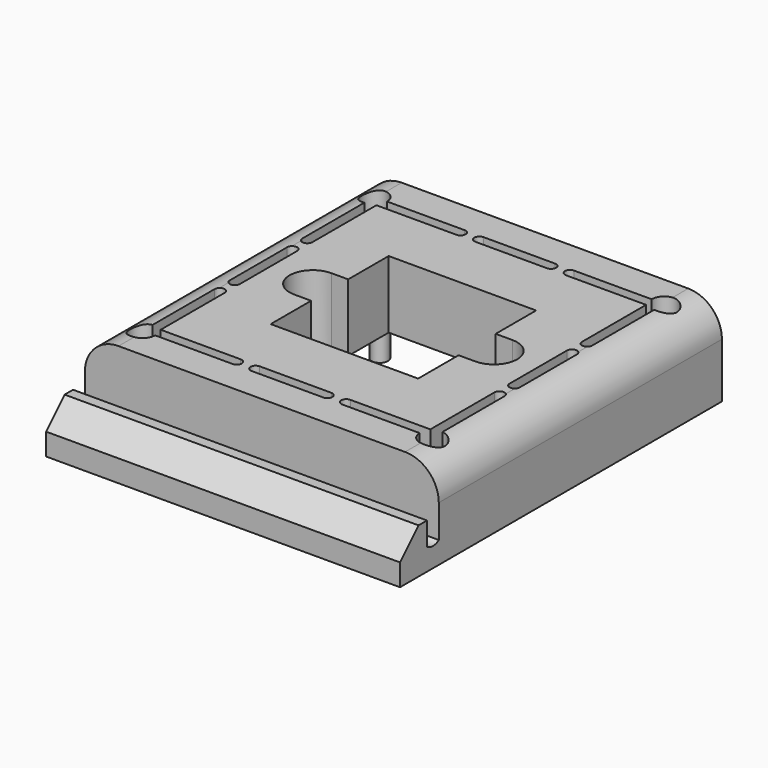
from build123d import *

# Parameters (mm, degrees)
F0_W        = 39
F0_H        = 39
F0_R        = 0.975
F1_DEPTH    = 9
F2_T1_DEPTH = 62
F4_DEPTH    = 21
F5_DEPTH    = 21
F6_DEPTH    = 5.5
F7_DEPTH    = 1.5
F8_DEPTH    = 2.5
F9_DEPTH    = 1.5
F10_R       = 1.25
F11_DEPTH   = 2.5
F12_DEPTH   = 5
F13_DEPTH   = 1


# Not quite as in the source:
# - a fillet or chamfer that OpenCascade refuses, or shapes differently, is made with other operations: its cross-section is extruded or revolved along the edge and cut away or added


with BuildPart() as f1:
    # F0 (on Top) → F1 (new body)
    with BuildSketch(Plane.XY):
        Polygon((-2.625, 21), (-21, 21), (-21, -21), (-2.625, -21), (2.625, -21), (21, -21), (21, 21), (2.625, 21), align=None)
        Rectangle(F0_W, F0_H, mode=Mode.SUBTRACT)
        Rectangle(F0_W, F0_H)
        with BuildLine():
            ThreePointArc((16, 4.25), (16.6, 4.85), (17.2, 4.25))
            Line((17.2, 4.25), (17.2, -4.25))
            ThreePointArc((17.2, -4.25), (16.6, -4.85), (16, -4.25))
            Line((16, -4.25), (16, -6.5))
            ThreePointArc((16, -6.5), (16.6, -5.9), (17.2, -6.5))
            Line((17.2, -6.5), (17.2, -15.7))
            ThreePointArc((17.2, -15.7), (18.2606601718, -18.2606601718), (15.7, -17.2))
            Line((15.7, -17.2), (6.5, -17.2))
            ThreePointArc((6.5, -17.2), (5.9, -16.6), (6.5, -16))
            Line((6.5, -16), (4.25, -16))
            ThreePointArc((4.25, -16), (4.85, -16.6), (4.25, -17.2))
            Line((4.25, -17.2), (-4.25, -17.2))
            ThreePointArc((-4.25, -17.2), (-4.85, -16.6), (-4.25, -16))
            Line((-4.25, -16), (-6.5, -16))
            ThreePointArc((-6.5, -16), (-5.9, -16.6), (-6.5, -17.2))
            Line((-6.5, -17.2), (-15.7, -17.2))
            ThreePointArc((-15.7, -17.2), (-18.2606601718, -18.2606601718), (-17.2, -15.7))
            Line((-17.2, -15.7), (-17.2, -6.5))
            ThreePointArc((-17.2, -6.5), (-16.6, -5.9), (-16, -6.5))
            Line((-16, -6.5), (-16, -4.25))
            ThreePointArc((-16, -4.25), (-16.6, -4.85), (-17.2, -4.25))
            Line((-17.2, -4.25), (-17.2, 4.25))
            ThreePointArc((-17.2, 4.25), (-16.6, 4.85), (-16, 4.25))
            Line((-16, 4.25), (-16, 6.5))
            ThreePointArc((-16, 6.5), (-16.6, 5.9), (-17.2, 6.5))
            Line((-17.2, 6.5), (-17.2, 15.7))
            ThreePointArc((-17.2, 15.7), (-18.2606601718, 18.2606601718), (-15.7, 17.2))
            Line((-15.7, 17.2), (-6.5, 17.2))
            ThreePointArc((-6.5, 17.2), (-5.9, 16.6), (-6.5, 16))
            Line((-6.5, 16), (-4.25, 16))
            ThreePointArc((-4.25, 16), (-4.85, 16.6), (-4.25, 17.2))
            Line((-4.25, 17.2), (4.25, 17.2))
            ThreePointArc((4.25, 17.2), (4.85, 16.6), (4.25, 16))
            Line((4.25, 16), (6.5, 16))
            ThreePointArc((6.5, 16), (5.9, 16.6), (6.5, 17.2))
            Line((6.5, 17.2), (15.7, 17.2))
            ThreePointArc((15.7, 17.2), (18.2606601718, 18.2606601718), (17.2, 15.7))
            Line((17.2, 15.7), (17.2, 6.5))
            ThreePointArc((17.2, 6.5), (16.6, 5.9), (16, 6.5))
            Line((16, 6.5), (16, 4.25))
        make_face(mode=Mode.SUBTRACT)
        Polygon((16, -4.25), (16, 4.25), (16, 6.5), (16, 16), (6.5, 16), (4.25, 16), (-4.25, 16), (-6.5, 16), (-16, 16), (-16, 6.5), (-16, 4.25), (-16, -4.25), (-16, -6.5), (-16, -16), (-6.5, -16), (-4.25, -16), (4.25, -16), (6.5, -16), (16, -16), (16, -6.5), align=None)
        with Locations((-14, -14)):
            Circle(F0_R, mode=Mode.SUBTRACT)
        with Locations((14, -14)):
            Circle(F0_R, mode=Mode.SUBTRACT)
        with Locations((-14, 14)):
            Circle(F0_R, mode=Mode.SUBTRACT)
        Polygon((-8.75, 14), (0, 14), (0, 10.75), (-8.75, 10.75), (-9.75, 10.75), (-9.75, 14), align=None, mode=Mode.SUBTRACT)
        with BuildLine():
            Line((-8.75, 8.75), (8.75, 8.75))
            Line((8.75, 8.75), (8.75, 2.75))
            Line((8.75, 2.75), (10.75, 2.75))
            ThreePointArc((10.75, 2.75), (13.5, 0), (10.75, -2.75))
            Line((10.75, -2.75), (8.75, -2.75))
            Line((8.75, -2.75), (8.75, -8.75))
            Line((8.75, -8.75), (-8.75, -8.75))
            Line((-8.75, -8.75), (-8.75, -2.75))
            Line((-8.75, -2.75), (-10.75, -2.75))
            ThreePointArc((-10.75, -2.75), (-13.5, 0), (-10.75, 2.75))
            Line((-10.75, 2.75), (-8.75, 2.75))
            Line((-8.75, 2.75), (-8.75, 8.75))
        make_face(mode=Mode.SUBTRACT)
        Polygon((10.75, 3.8126846775), (10.75, 8.75), (10.75, 9.75), (14, 9.75), (14, 8.75), (14, 3.8126846775), align=None, mode=Mode.SUBTRACT)
        with Locations((14, 14)):
            Circle(F0_R, mode=Mode.SUBTRACT)
        Polygon((0, 10.75), (0, 14), (-8.75, 14), (-9.75, 14), (-9.75, 10.75), (-8.75, 10.75), align=None)
        Polygon((10.75, 9.75), (10.75, 8.75), (10.75, 3.8126846775), (14, 3.8126846775), (14, 8.75), (14, 9.75), align=None)
        with Locations((14, -14)):
            Circle(F0_R)
        with Locations((-14, -14)):
            Circle(F0_R)
        with Locations((-14, 14)):
            Circle(F0_R)
        with Locations((14, 14)):
            Circle(F0_R)
    extrude(amount=F1_DEPTH)

    # F2: fillet of radius 4 on 2 edges, made by hand

    # F2_s2 → F2_t1 (cut)
    with BuildSketch(Plane.XZ.offset(-31)):
        with BuildLine():
            ThreePointArc((-21, 5), (-19.8284271247, 7.8284271247), (-17, 9))
            Line((-17, 9), (-21, 9))
            Line((-21, 9), (-21, 5))
        make_face()
        with BuildLine():
            ThreePointArc((21, 5), (19.8284271247, 7.8284271247), (17, 9))
            Line((17, 9), (21, 9))
            Line((21, 9), (21, 5))
        make_face()
    extrude(amount=F2_T1_DEPTH, mode=Mode.SUBTRACT)

    # F3 (on Right) → F4 (join)
    with BuildSketch(Plane.YZ):
        with BuildLine():
            Line((-21, 0), (-21, 1.1))
            ThreePointArc((-21, 1.1), (-21.875, 0.8183492931), (-22.75, 1.1))
            Line((-22.75, 1.1), (-22.75, 3.85))
            Line((-22.75, 3.85), (-24, 3.85))
            Line((-24, 3.85), (-26.75, 1.1))
            Line((-26.75, 1.1), (-26.75, -1.5))
            Line((-26.75, -1.5), (-22.75, -1.5))
            Line((-22.75, -1.5), (-21, -1.5))
            Line((-21, -1.5), (-21, 0))
        make_face()
    extrude(amount=F4_DEPTH)

    # F5 (add): a face of the model
    f5_faces = [f1.faces().sort_by_distance(p)[0] for p in [
        (0, -24.00739598, 0.5868334208),
    ]]
    extrude(f5_faces, amount=F5_DEPTH)

    # F0 (on Top) → F6 (join)
    with BuildSketch(Plane.XY):
        with Locations((-14, -14)):
            Circle(F0_R)
        with Locations((14, -14)):
            Circle(F0_R)
        with Locations((-14, 14)):
            Circle(F0_R)
        with Locations((14, 14)):
            Circle(F0_R)
    extrude(amount=-F6_DEPTH)

    # F0 (on Top) → F7 (join)
    with BuildSketch(Plane.XY):
        Rectangle(F0_W, F0_H)
        with BuildLine():
            ThreePointArc((16, 4.25), (16.6, 4.85), (17.2, 4.25))
            Line((17.2, 4.25), (17.2, -4.25))
            ThreePointArc((17.2, -4.25), (16.6, -4.85), (16, -4.25))
            Line((16, -4.25), (16, -6.5))
            ThreePointArc((16, -6.5), (16.6, -5.9), (17.2, -6.5))
            Line((17.2, -6.5), (17.2, -15.7))
            ThreePointArc((17.2, -15.7), (18.2606601718, -18.2606601718), (15.7, -17.2))
            Line((15.7, -17.2), (6.5, -17.2))
            ThreePointArc((6.5, -17.2), (5.9, -16.6), (6.5, -16))
            Line((6.5, -16), (4.25, -16))
            ThreePointArc((4.25, -16), (4.85, -16.6), (4.25, -17.2))
            Line((4.25, -17.2), (-4.25, -17.2))
            ThreePointArc((-4.25, -17.2), (-4.85, -16.6), (-4.25, -16))
            Line((-4.25, -16), (-6.5, -16))
            ThreePointArc((-6.5, -16), (-5.9, -16.6), (-6.5, -17.2))
            Line((-6.5, -17.2), (-15.7, -17.2))
            ThreePointArc((-15.7, -17.2), (-18.2606601718, -18.2606601718), (-17.2, -15.7))
            Line((-17.2, -15.7), (-17.2, -6.5))
            ThreePointArc((-17.2, -6.5), (-16.6, -5.9), (-16, -6.5))
            Line((-16, -6.5), (-16, -4.25))
            ThreePointArc((-16, -4.25), (-16.6, -4.85), (-17.2, -4.25))
            Line((-17.2, -4.25), (-17.2, 4.25))
            ThreePointArc((-17.2, 4.25), (-16.6, 4.85), (-16, 4.25))
            Line((-16, 4.25), (-16, 6.5))
            ThreePointArc((-16, 6.5), (-16.6, 5.9), (-17.2, 6.5))
            Line((-17.2, 6.5), (-17.2, 15.7))
            ThreePointArc((-17.2, 15.7), (-18.2606601718, 18.2606601718), (-15.7, 17.2))
            Line((-15.7, 17.2), (-6.5, 17.2))
            ThreePointArc((-6.5, 17.2), (-5.9, 16.6), (-6.5, 16))
            Line((-6.5, 16), (-4.25, 16))
            ThreePointArc((-4.25, 16), (-4.85, 16.6), (-4.25, 17.2))
            Line((-4.25, 17.2), (4.25, 17.2))
            ThreePointArc((4.25, 17.2), (4.85, 16.6), (4.25, 16))
            Line((4.25, 16), (6.5, 16))
            ThreePointArc((6.5, 16), (5.9, 16.6), (6.5, 17.2))
            Line((6.5, 17.2), (15.7, 17.2))
            ThreePointArc((15.7, 17.2), (18.2606601718, 18.2606601718), (17.2, 15.7))
            Line((17.2, 15.7), (17.2, 6.5))
            ThreePointArc((17.2, 6.5), (16.6, 5.9), (16, 6.5))
            Line((16, 6.5), (16, 4.25))
        make_face(mode=Mode.SUBTRACT)
    extrude(amount=-F7_DEPTH)

    # F8 (cut): a face of the model
    f8_faces = [f1.faces().sort_by_distance(p)[0] for p in [
        (-18.9484567107, 0, -1.5),
    ]]
    extrude(f8_faces, amount=-F8_DEPTH, mode=Mode.SUBTRACT)

    # F0 (on Top) → F9 (join)
    with BuildSketch(Plane.XY):
        Polygon((-2.625, 21), (-21, 21), (-21, -21), (-2.625, -21), (2.625, -21), (21, -21), (21, 21), (2.625, 21), align=None)
        Rectangle(F0_W, F0_H, mode=Mode.SUBTRACT)
    extrude(amount=-F9_DEPTH)

    # F10 (on face) → F11 (cut)
    with BuildSketch(Plane(origin=(0, 0, -1.5), x_dir=(1, 0, 0), z_dir=(0, 0, -1))):
        with Locations((10.5, 24.25)):
            Circle(F10_R)
        with Locations((0, 24.25)):
            Circle(F10_R)
        with Locations((-10.5, 24.25)):
            Circle(F10_R)
    extrude(amount=-F11_DEPTH, mode=Mode.SUBTRACT)

    # F0 (on Top) → F12 (cut)
    with BuildSketch(Plane.XY):
        Polygon((10.75, 9.75), (10.75, 8.75), (10.75, 3.8126846775), (14, 3.8126846775), (14, 8.75), (14, 9.75), align=None)
        Polygon((0, 10.75), (0, 14), (-8.75, 14), (-9.75, 14), (-9.75, 10.75), (-8.75, 10.75), align=None)
    extrude(amount=F12_DEPTH, mode=Mode.SUBTRACT)

    # F0 (on Top) → F13 (cut)
    with BuildSketch(Plane.XY):
        Polygon((16, -4.25), (16, 4.25), (16, 6.5), (16, 16), (6.5, 16), (4.25, 16), (-4.25, 16), (-6.5, 16), (-16, 16), (-16, 6.5), (-16, 4.25), (-16, -4.25), (-16, -6.5), (-16, -16), (-6.5, -16), (-4.25, -16), (4.25, -16), (6.5, -16), (16, -16), (16, -6.5), align=None)
        with Locations((-14, -14)):
            Circle(F0_R, mode=Mode.SUBTRACT)
        with Locations((14, -14)):
            Circle(F0_R, mode=Mode.SUBTRACT)
        with Locations((-14, 14)):
            Circle(F0_R, mode=Mode.SUBTRACT)
        Polygon((-8.75, 14), (0, 14), (0, 10.75), (-8.75, 10.75), (-9.75, 10.75), (-9.75, 14), align=None, mode=Mode.SUBTRACT)
        with BuildLine():
            Line((-8.75, 8.75), (8.75, 8.75))
            Line((8.75, 8.75), (8.75, 2.75))
            Line((8.75, 2.75), (10.75, 2.75))
            ThreePointArc((10.75, 2.75), (13.5, 0), (10.75, -2.75))
            Line((10.75, -2.75), (8.75, -2.75))
            Line((8.75, -2.75), (8.75, -8.75))
            Line((8.75, -8.75), (-8.75, -8.75))
            Line((-8.75, -8.75), (-8.75, -2.75))
            Line((-8.75, -2.75), (-10.75, -2.75))
            ThreePointArc((-10.75, -2.75), (-13.5, 0), (-10.75, 2.75))
            Line((-10.75, 2.75), (-8.75, 2.75))
            Line((-8.75, 2.75), (-8.75, 8.75))
        make_face(mode=Mode.SUBTRACT)
        Polygon((10.75, 3.8126846775), (10.75, 8.75), (10.75, 9.75), (14, 9.75), (14, 8.75), (14, 3.8126846775), align=None, mode=Mode.SUBTRACT)
        with Locations((14, 14)):
            Circle(F0_R, mode=Mode.SUBTRACT)
    extrude(amount=F13_DEPTH, mode=Mode.SUBTRACT)


solid = f1.part
